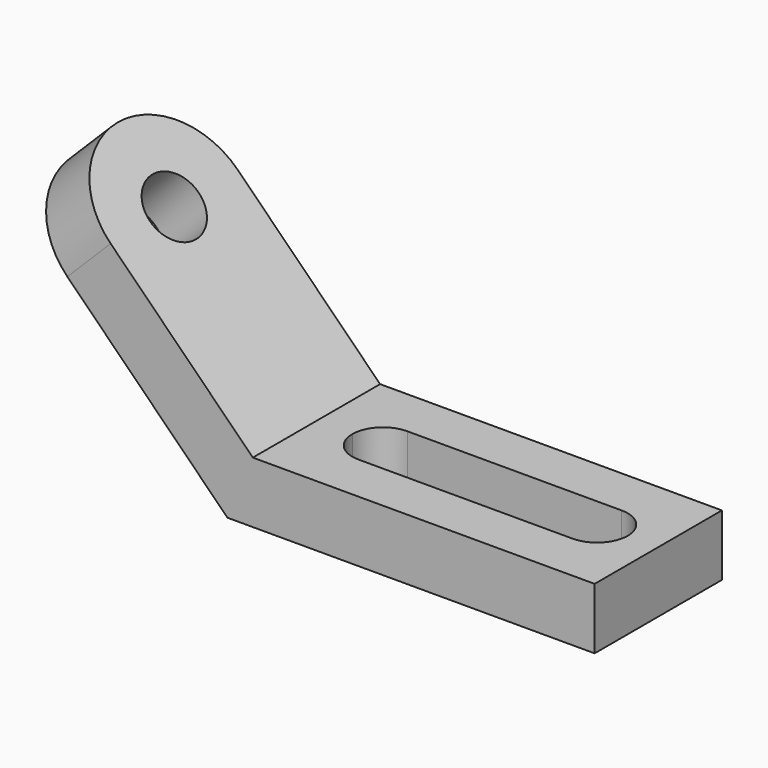
from build123d import *

# Parameters (mm, degrees)
F1_DEPTH = 52
F2_R     = 10
F3_DEPTH = 25
F4_R     = 25.99999
F6_DEPTH = 25
F7_R     = 9.99999


# Not quite as in the source:
# - a fillet or chamfer is up to 0.001 mm smaller than in the source, because OpenCascade refuses the exact size
# - a feature names something its author has since deleted; it is built from what else it names


with BuildPart() as f1:
    # F0 (on Front) → F1 (new body)
    with BuildSketch(Plane.XZ):
        Polygon((-120, 0), (0, 0), (0, 20), (-111.7157287525, 20), (-176.5685424949, 84.8528137424), (-190.7106781187, 70.7106781187), align=None)
    extrude(amount=F1_DEPTH)

    # F2 (on face) → F3 (cut)
    with BuildSketch(Plane(origin=(-45.8578643763, 0, -45.8578643763), x_dir=(0.7071067812, 0, -0.7071067812), z_dir=(0.7071067812, 0, 0.7071067812))):
        with Locations((-158.8528137424, -26)):
            Circle(F2_R)
    extrude(amount=-F3_DEPTH, mode=Mode.SUBTRACT)

    # F4 (radius 26 in the source; OpenCascade refuses exactly that, so slightly less here)
    f4_edges = [f1.edges().sort_by_distance(p)[0] for p in [
        (-183.63961, 0, 77.781746),
        (-183.63961, -52, 77.781746),
    ]]
    fillet(f4_edges, radius=F4_R)

    # F5 (on face) → F6 (cut)
    with BuildSketch(Plane.XY.offset(20)):
        Polygon((-10, -16), (-100, -16), (-100, -26), (-100, -36), (-10, -36), (-10, -26), align=None)
    extrude(amount=-F6_DEPTH, mode=Mode.SUBTRACT)

    # F7 (radius 10 in the source; OpenCascade refuses exactly that, so slightly less here)
    f7_edges = [f1.edges().sort_by_distance(p)[0] for p in [
        (-10, -16, 10),
        (-10, -36, 10),
        (-100, -16, 10),
        (-100, -36, 10),
    ]]
    fillet(f7_edges, radius=F7_R)


solid = f1.part
